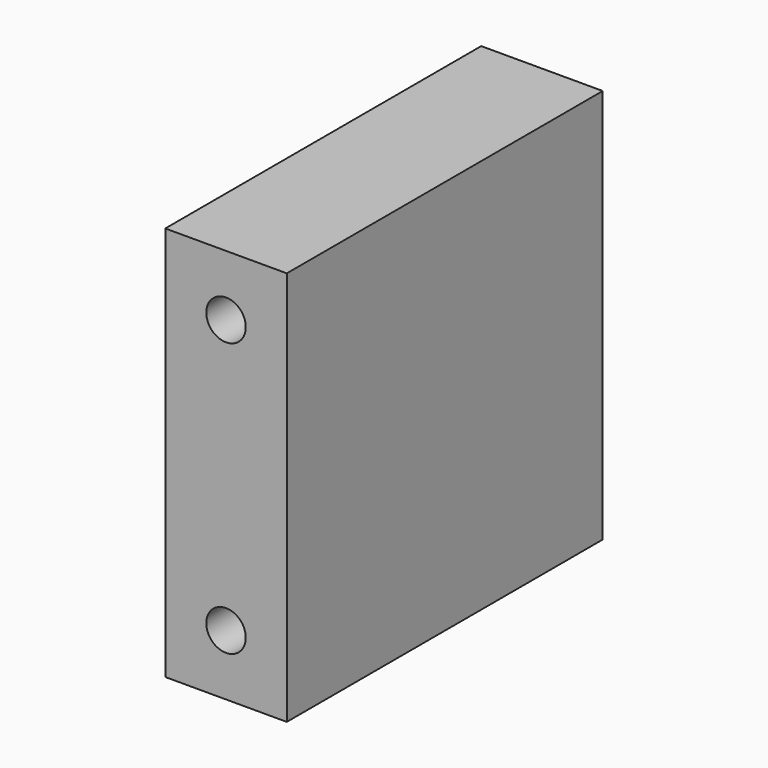
from build123d import *

# Parameters (mm, degrees)
F1_DEPTH = 65


# Not quite as in the source:
# - a feature names something its author has since deleted; it is built from what else it names


with BuildPart() as f1:
    # F0 (on Front) → F1 (new body)
    with BuildSketch(Plane.XZ):
        Polygon((0, 10), (0, 0), (20, 0), (20, 65), (0, 65), (0, 55), align=None)
        with BuildLine():
            ThreePointArc((13.25, 10), (10, 6.75), (6.75, 10))
            ThreePointArc((6.75, 10), (10, 13.25), (13.25, 10))
        make_face(mode=Mode.SUBTRACT)
        with BuildLine():
            ThreePointArc((13.25, 55), (10, 51.75), (6.75, 55))
            ThreePointArc((6.75, 55), (10, 58.25), (13.25, 55))
        make_face(mode=Mode.SUBTRACT)
    extrude(amount=F1_DEPTH)


solid = f1.part
